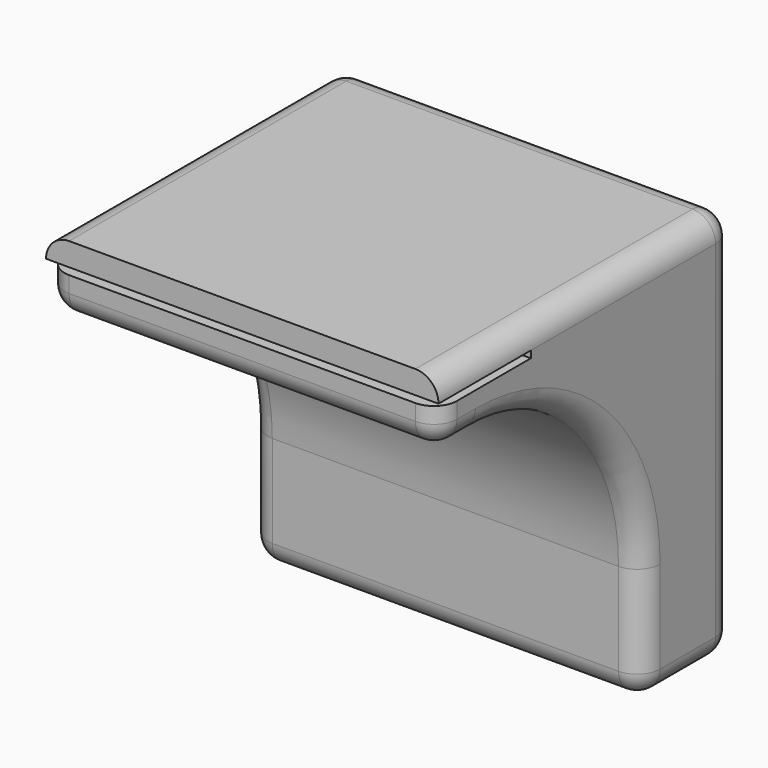
from build123d import *

# Parameters (mm, degrees)
F1_DEPTH  = 60
F2_DEPTH  = 85
F3_W      = 65
F3_H      = 20
F4_DEPTH  = 10
F5_W      = 65
F5_H      = 20
F6_DEPTH  = 10
F9_W      = 85
F9_H      = 25
F10_DEPTH = 1.5
F11_F1_R  = 5
F11_F2_R  = 5
F12_W     = 85
F12_H     = 60
F13_DEPTH = 70
F14_R     = 45
F15_R     = 4.99999
F16_R     = 4.99999
F17_W     = 85
F17_H     = 1.5
F18_DEPTH = 5
F19_W     = 85
F19_H     = 5
F20_DEPTH = 5
F21_W     = 5
F21_H     = 10
F22_DEPTH = 85
F23_R     = 4.99999


# Not quite as in the source:
# - a fillet or chamfer is up to 0.001 mm smaller than in the source, because OpenCascade refuses the exact size


with BuildPart() as f1:
    # F0 (on Top) → F1 (new body)
    with BuildSketch(Plane.XY):
        Polygon((-61.8206309527, 56.9930104911), (-61.8206309527, -28.0069895089), (23.1793690473, -28.0069895089), (23.1793690473, 56.9930104911), (13.1793690473, 56.9930104911), (13.1793690473, 36.9930104911), (-51.8206309527, 36.9930104911), (-51.8206309527, 56.9930104911), align=None)
    extrude(amount=F1_DEPTH)

    # F0 (on Top) → F2 (join)
    with BuildSketch(Plane.XY):
        Polygon((-61.8206309527, 56.9930104911), (-61.8206309527, -28.0069895089), (23.1793690473, -28.0069895089), (23.1793690473, 56.9930104911), (13.1793690473, 56.9930104911), (13.1793690473, 36.9930104911), (-51.8206309527, 36.9930104911), (-51.8206309527, 56.9930104911), align=None)
    extrude(amount=F2_DEPTH)

    # F3 (on face) → F4 (join)
    with BuildSketch(Plane.XY.offset(85)):
        with Locations((-19.3206309527, 46.9930104911)):
            Rectangle(F3_W, F3_H)
    extrude(amount=-F4_DEPTH)

    # F5 (on face) → F6 (join)
    with BuildSketch(Plane(origin=(0, 0, 0), x_dir=(1, 0, 0), z_dir=(0, 0, -1))):
        with Locations((-19.3206309527, -46.9930104911)):
            Rectangle(F5_W, F5_H)
    extrude(amount=-F6_DEPTH)

    # F9 (on offset) → F10 (cut)
    with BuildSketch(Plane.XY.offset(80)):
        with Locations((-19.3206309527, -15.5069895089)):
            Rectangle(F9_W, F9_H)
    extrude(amount=-F10_DEPTH, mode=Mode.SUBTRACT)

    # F11: fillet of radius 5 on 4 edges, made by hand

    # F11_f1
    f11_f1_edges = [f1.edges().sort_by_distance(p)[0] for p in [
        (13.1793690473, 46.9930104911, 10),
        (-19.3206309527, 36.9930104911, 10),
        (-51.8206309527, 46.9930104911, 10),
    ]]
    fillet(f11_f1_edges, radius=F11_F1_R)

    # F11_f2
    f11_f2_edges = [f1.edges().sort_by_distance(p)[0] for p in [
        (-19.3206309527, 56.9930104911, 10),
        (-50.3561648586, 56.9930104911, 11.4644660941),
        (11.7149029532, 56.9930104911, 11.4644660941),
    ]]
    fillet(f11_f2_edges, radius=F11_F2_R)

    # F12 (on face) → F13 (cut)
    with BuildSketch(Plane(origin=(0, 0, 0), x_dir=(1, 0, 0), z_dir=(0, 0, -1))):
        with Locations((-19.3206309527, -1.9930104911)):
            Rectangle(F12_W, F12_H)
    extrude(amount=-F13_DEPTH, mode=Mode.SUBTRACT)

    # F14
    f14_edges = [f1.edges().sort_by_distance(p)[0] for p in [
        (-19.320631, 31.99301, 70),
    ]]
    fillet(f14_edges, radius=F14_R)

    # F15 (radius 5 in the source; OpenCascade refuses exactly that, so slightly less here)
    f15_edges = [f1.edges().sort_by_distance(p)[0] for p in [
        (-19.320631, 56.99301, 0),
        (-61.820631, 56.99301, 42.5),
        (23.179369, 56.99301, 42.5),
        (-61.820631, 44.49301, 0),
        (23.179369, 44.49301, 0),
        (-19.320631, 31.99301, 0),
        (-61.820631, -20.50699, 70),
        (23.179369, 18.812816, 56.819805),
        (-61.820631, 31.99301, 12.5),
        (-61.820631, 18.812816, 56.819805),
        (-61.820631, 14.49301, 85),
        (23.179369, 31.99301, 12.5),
        (23.179369, -20.50699, 70),
        (-19.320631, 56.99301, 85),
        (23.179369, 14.49301, 85),
    ]]
    fillet(f15_edges, radius=F15_R)

    # F16 (radius 5 in the source; OpenCascade refuses exactly that, so slightly less here)
    f16_edges = [f1.edges().sort_by_distance(p)[0] for p in [
        (-19.320631, 51.99302, 0),
        (18.179379, 44.49301, 0),
        (-56.820641, 44.49301, 0),
        (-19.320631, 36.993, 0),
        (-19.320631, -28.00699, 70),
    ]]
    fillet(f16_edges, radius=F16_R)

    # F17 (on face) → F18 (cut)
    with BuildSketch(Plane.XZ.offset(3.0069895089)):
        with Locations((-19.3206309527, 79.25)):
            Rectangle(F17_W, F17_H)
    extrude(amount=-F18_DEPTH, mode=Mode.SUBTRACT)

    # F19 (on face) → F20 (cut)
    with BuildSketch(Plane.XZ.offset(28.0069895089)):
        with Locations((-19.3206309527, 82.5)):
            Rectangle(F19_W, F19_H)
    extrude(amount=-F20_DEPTH, mode=Mode.SUBTRACT)

    # F21 (on face) → F22 (cut)
    with BuildSketch(Plane(origin=(-61.8206309527, 0, 0), x_dir=(0, -1, 0), z_dir=(-1, 0, 0))):
        with Locations((25.5069895089, 73.5)):
            Rectangle(F21_W, F21_H)
    extrude(amount=-F22_DEPTH, mode=Mode.SUBTRACT)

    # F23 (radius 5 in the source; OpenCascade refuses exactly that, so slightly less here)
    f23_edges = [f1.edges().sort_by_distance(p)[0] for p in [
        (-19.320631, -23.00699, 70),
        (-61.820631, -23.00699, 76.749995),
        (-60.356168, -23.00699, 71.464463),
        (21.714906, -23.00699, 71.464463),
        (23.179369, -23.00699, 76.749995),
    ]]
    fillet(f23_edges, radius=F23_R)


solid = f1.part
